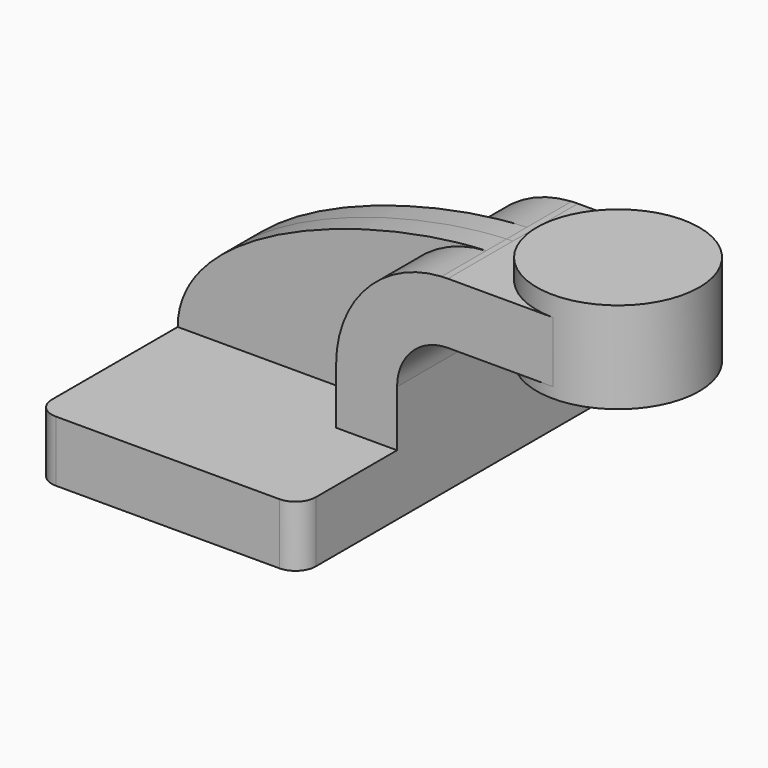
from build123d import *

# Parameters (mm, degrees)
F1_DEPTH = 63.5
F2_DEPTH = 7.9375
F3_DEPTH = 25.4
F5_R     = 6.35


# Not quite as in the source:
# - a feature names something its author has since deleted; it is built from what else it names


with BuildPart() as f1:
    # F0 (on Front) → F1 (new body, symmetric)
    with BuildSketch(Plane.XZ):
        Polygon((-41.275, 9.525), (-41.275, -9.525), (41.275, -9.525), (41.275, 9.525), (22.225, 9.525), align=None)
    extrude(amount=F1_DEPTH, both=True)

    # F0 (on Front) → F2 (join, symmetric)
    with BuildSketch(Plane.XZ):
        with BuildLine():
            add(Edge.make_bspline(
                [(-41.275, 9.525), (-41.112587778, 40.4556006324), (19.5290392467, 60.5257095831), (55.1792354288, 61.8695520445)],
                knots=[0, 0, 0, 0, 109.4601917253, 109.4601917253, 109.4601917253, 109.4601917253], degree=3))
            Line((-41.275, 9.525), (22.225, 9.525))
            Line((22.225, 9.525), (22.225, 27.0002))
            ThreePointArc((22.225, 27.0002), (31.7670866758, 50.9890168982), (55.1792354288, 61.8695520445))
        make_face()
    extrude(amount=F2_DEPTH, both=True)

    # F0 (on Front) → F3 (join, symmetric)
    with BuildSketch(Plane.XZ):
        with BuildLine():
            Line((22.225, 9.525), (41.275, 9.525))
            Line((41.275, 9.525), (41.275, 27.0002))
            ThreePointArc((41.275, 27.0002), (45.9246798487, 38.2255201513), (57.15, 42.8752))
            Line((57.15, 42.8752), (90.0369858318, 42.8752))
            Line((90.0369858318, 42.8752), (90.0369858318, 61.9252))
            Line((90.0369858318, 61.9252), (57.15, 61.9252))
            add(Edge.make_bspline(
                [(55.1792354288, 61.8695520445), (55.8450599549, 61.8946504554), (56.5021670835, 61.9132168549), (57.15, 61.9252)],
                knots=[109.4601917253, 109.4601917253, 109.4601917253, 109.4601917253, 111.5045361635, 111.5045361635, 111.5045361635, 111.5045361635], degree=3))
            ThreePointArc((55.1792354288, 61.8695520445), (31.7670866758, 50.9890168982), (22.225, 27.0002))
            Line((22.225, 27.0002), (22.225, 9.525))
        make_face()
    extrude(amount=F3_DEPTH, both=True)

    # F0 (on Front) → F4 (revolve)
    with BuildSketch(Plane.XZ):
        Polygon((90.0369858318, 68.1490233362), (90.0369858318, 61.9252), (90.0369858318, 42.8752), (90.0369858318, 39.5740233362), (115.4369858318, 39.5740233362), (115.4369858318, 68.1490233362), align=None)
    revolve(axis=Axis((90.0369858318, 0, 53.8615233362), (0, 0, -1)))

    # F5
    f5_edges = [f1.edges().sort_by_distance(p)[0] for p in [
        (-41.275, -63.5, 0),
        (41.275, -63.5, 0),
        (41.275, 63.5, 0),
        (-41.275, 63.5, 0),
    ]]
    fillet(f5_edges, radius=F5_R)


solid = f1.part
